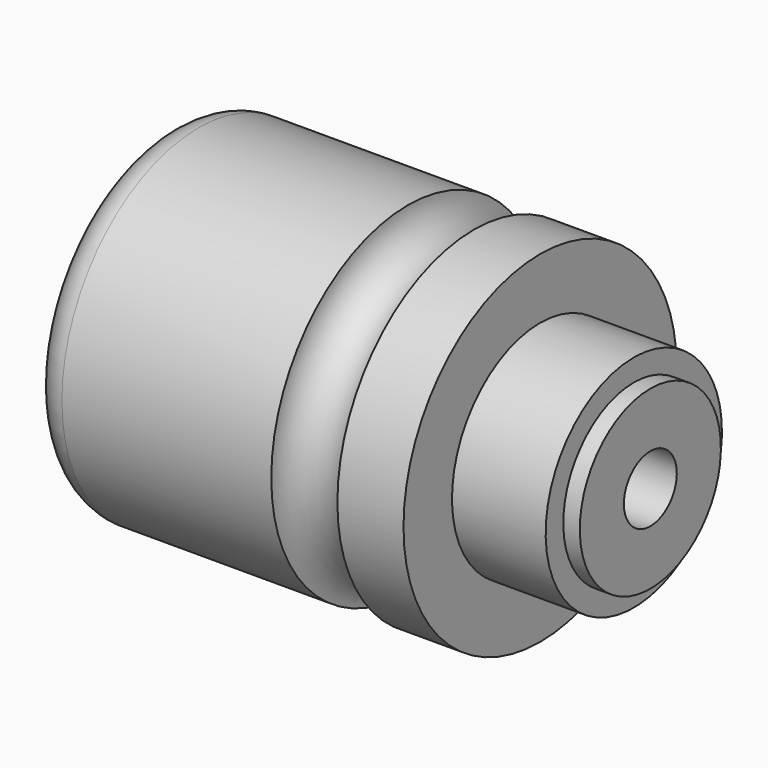
from build123d import *

# Parameters (mm, degrees)
F4_R = 5.99999


# Not quite as in the source:
# - a fillet or chamfer is up to 0.001 mm smaller than in the source, because OpenCascade refuses the exact size


with BuildPart() as f1:
    # F0 (on Front) → F1 (revolve)
    with BuildSketch(Plane.XZ):
        with BuildLine():
            Line((0, 31), (0, 0))
            Line((0, 0), (88, 0))
            Line((88, 0), (88, 16))
            Line((88, 16), (85, 16))
            Line((85, 16), (85, 20))
            Line((85, 20), (68, 20))
            Line((68, 20), (68, 31))
            Line((68, 31), (56, 31))
            ThreePointArc((56, 31), (50, 25), (44, 31))
            Line((44, 31), (0, 31))
        make_face()
    revolve(axis=Axis((55.6183233857, 0, 0), (1, 0, 0)))

    # F2 (on Front) → F3 (revolve, cut)
    with BuildSketch(Plane.XZ):
        Polygon((0, 25), (0, 0), (88, 0), (88, 6), (30, 6), (30, 16), (22, 16), (22, 20.5), (15, 20.5), (15, 12.5), (12, 12.5), (12, 16), (1.5, 16), (1.5, 25), align=None)
    revolve(axis=Axis((-12.6493745584, 0, 0), (-1, 0, 0)), mode=Mode.SUBTRACT)

    # F4 (radius 6 in the source; OpenCascade refuses exactly that, so slightly less here)
    f4_edges = [f1.edges().sort_by_distance(p)[0] for p in [
        (0, 0, -31),
    ]]
    fillet(f4_edges, radius=F4_R)


solid = f1.part
